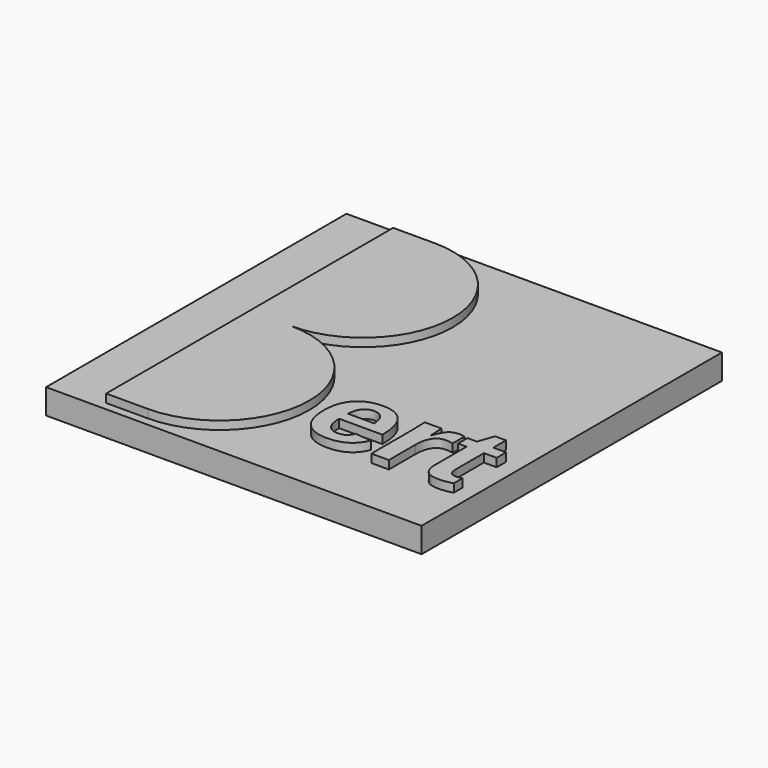
from build123d import *

# Parameters (mm, degrees)
F0_W         = 45
F0_H         = 45
F0_TEXT_SIZE = 15.2777777778
F1_DEPTH     = 3
F2_DEPTH     = 1


# Not quite as in the source:
# - Text() gives the source's letters only with a copy of the font that has no kerning and outlines rounded to 1/6400 em; it was checked with that copy


with BuildPart() as f1:
    # F0 (on Top) → F1 (new body)
    with BuildSketch(Plane.XY):
        with Locations((-17.3771874607, -9.7084985673)):
            Rectangle(F0_W, F0_H)
        with BuildLine():
            add(Edge.make_bspline(
                [(-8.1976327438, -23.1650957896), (-9.0570077438, -25.3588891923), (-11.6828757994, -25.3588891923)],
                knots=[0, 0, 0, 1, 1, 1], degree=2))
            add(Edge.make_bspline(
                [(-11.6828757994, -25.3588891923), (-13.5018862161, -25.3588891923), (-14.4794252786, -24.2798961368)],
                knots=[0, 0, 0, 1, 1, 1], degree=2))
            add(Edge.make_bspline(
                [(-14.4794252786, -24.2798961368), (-15.4569643411, -23.2009030812), (-15.4569643411, -21.1360159285)],
                knots=[0, 0, 0, 1, 1, 1], degree=2))
            add(Edge.make_bspline(
                [(-15.4569643411, -21.1360159285), (-15.4569643411, -19.1355819007), (-14.4651023619, -18.0613631507)],
                knots=[0, 0, 0, 1, 1, 1], degree=2))
            add(Edge.make_bspline(
                [(-14.4651023619, -18.0613631507), (-13.4732403827, -16.9871444007), (-11.6518428133, -16.9871444007)],
                knots=[0, 0, 0, 1, 1, 1], degree=2))
            add(Edge.make_bspline(
                [(-11.6518428133, -16.9871444007), (-9.9139955911, -16.9871444007), (-8.996135348, -18.1401391923)],
                knots=[0, 0, 0, 1, 1, 1], degree=2))
            add(Edge.make_bspline(
                [(-8.996135348, -18.1401391923), (-8.078275105, -19.293133984), (-8.078275105, -21.5155732201)],
                knots=[0, 0, 0, 1, 1, 1], degree=2))
            Line((-8.078275105, -21.5155732201), (-8.078275105, -21.5752520396))
            Line((-8.078275105, -21.5752520396), (-13.25600948, -21.5752520396))
            add(Edge.make_bspline(
                [(-13.25600948, -21.5752520396), (-13.25600948, -22.7545055118), (-12.8191605216, -23.3548744354)],
                knots=[0, 0, 0, 1, 1, 1], degree=2))
            add(Edge.make_bspline(
                [(-12.8191605216, -23.3548744354), (-12.3823115633, -23.955243359), (-11.5778410772, -23.955243359)],
                knots=[0, 0, 0, 1, 1, 1], degree=2))
            add(Edge.make_bspline(
                [(-11.5778410772, -23.955243359), (-10.4654278827, -23.955243359), (-10.1741952438, -22.9932207896)],
                knots=[0, 0, 0, 1, 1, 1], degree=2))
            Line((-10.1741952438, -22.9932207896), (-8.1976327438, -23.1650957896))
        make_face(mode=Mode.SUBTRACT)
        with BuildLine():
            Line((-4.3948983688, -25.2084985673), (-6.4908185077, -25.2084985673))
            Line((-6.4908185077, -25.2084985673), (-6.4908185077, -19.0305471785))
            add(Edge.make_bspline(
                [(-6.4908185077, -19.0305471785), (-6.4908185077, -18.3669187062), (-6.50991573, -17.9229082896)],
                knots=[0, 0, 0, 1, 1, 1], degree=2))
            add(Edge.make_bspline(
                [(-6.50991573, -17.9229082896), (-6.5290129522, -17.4788978729), (-6.5504973272, -17.1375350257)],
                knots=[0, 0, 0, 1, 1, 1], degree=2))
            Line((-6.5504973272, -17.1375350257), (-4.5524504522, -17.1375350257))
            add(Edge.make_bspline(
                [(-4.5524504522, -17.1375350257), (-4.5285789244, -17.2712155812), (-4.4915780563, -17.9539412757)],
                knots=[0, 0, 0, 1, 1, 1], degree=2))
            add(Edge.make_bspline(
                [(-4.4915780563, -17.9539412757), (-4.4545771883, -18.6366669701), (-4.4545771883, -18.8610593312)],
                knots=[0, 0, 0, 1, 1, 1], degree=2))
            Line((-4.4545771883, -18.8610593312), (-4.4235442022, -18.8610593312))
            add(Edge.make_bspline(
                [(-4.4235442022, -18.8610593312), (-4.1179886466, -18.0088457896), (-3.8792733688, -17.6627086368)],
                knots=[0, 0, 0, 1, 1, 1], degree=2))
            add(Edge.make_bspline(
                [(-3.8792733688, -17.6627086368), (-3.6405580911, -17.316571484), (-3.3123245841, -17.1482772132)],
                knots=[0, 0, 0, 1, 1, 1], degree=2))
            add(Edge.make_bspline(
                [(-3.3123245841, -17.1482772132), (-2.9840910772, -16.9799829423), (-2.492337605, -16.9799829423)],
                knots=[0, 0, 0, 1, 1, 1], degree=2))
            add(Edge.make_bspline(
                [(-2.492337605, -16.9799829423), (-2.0889087855, -16.9799829423), (-1.8430320494, -17.0921791229)],
                knots=[0, 0, 0, 1, 1, 1], degree=2))
            Line((-1.8430320494, -17.0921791229), (-1.8430320494, -18.8443492618))
            add(Edge.make_bspline(
                [(-1.8430320494, -18.8443492618), (-2.3514955911, -18.7321530812), (-2.7382143411, -18.7321530812)],
                knots=[0, 0, 0, 1, 1, 1], degree=2))
            add(Edge.make_bspline(
                [(-2.7382143411, -18.7321530812), (-3.5212004522, -18.7321530812), (-3.9580494105, -19.3671357201)],
                knots=[0, 0, 0, 1, 1, 1], degree=2))
            add(Edge.make_bspline(
                [(-3.9580494105, -19.3671357201), (-4.3948983688, -20.002118359), (-4.3948983688, -21.248212109)],
                knots=[0, 0, 0, 1, 1, 1], degree=2))
            Line((-4.3948983688, -21.248212109), (-4.3948983688, -25.2084985673))
        make_face(mode=Mode.SUBTRACT)
        with BuildLine():
            add(Edge.make_bspline(
                [(3.2893464228, -25.0891409285), (2.51352177, -25.3421791229), (1.5228533673, -25.3421791229)],
                knots=[0, 0, 0, 1, 1, 1], degree=2))
            add(Edge.make_bspline(
                [(1.5228533673, -25.3421791229), (0.5966380895, -25.3421791229), (0.0965295825, -24.8384898868)],
                knots=[0, 0, 0, 1, 1, 1], degree=2))
            add(Edge.make_bspline(
                [(0.0965295825, -24.8384898868), (-0.4035789244, -24.3348006507), (-0.4035789244, -23.3130992618)],
                knots=[0, 0, 0, 1, 1, 1], degree=2))
            Line((-0.4035789244, -23.3130992618), (-0.4035789244, -18.5531166229))
            Line((-0.4035789244, -18.5531166229), (-1.4252803133, -18.5531166229))
            Line((-1.4252803133, -18.5531166229), (-1.4252803133, -17.1375350257))
            Line((-1.4252803133, -17.1375350257), (-0.2985442022, -17.1375350257))
            Line((-0.2985442022, -17.1375350257), (0.3579228117, -15.2421357201))
            Line((0.3579228117, -15.2421357201), (1.6708568395, -15.2421357201))
            Line((1.6708568395, -15.2421357201), (1.6708568395, -17.1375350257))
            Line((1.6708568395, -17.1375350257), (3.20102177, -17.1375350257))
            Line((3.20102177, -17.1375350257), (3.20102177, -18.5531166229))
            Line((3.20102177, -18.5531166229), (1.6708568395, -18.5531166229))
            Line((1.6708568395, -18.5531166229), (1.6708568395, -22.7473440535))
            add(Edge.make_bspline(
                [(1.6708568395, -22.7473440535), (1.6708568395, -23.3369707896), (1.8952492006, -23.6162676646)],
                knots=[0, 0, 0, 1, 1, 1], degree=2))
            add(Edge.make_bspline(
                [(1.8952492006, -23.6162676646), (2.1196415617, -23.8955645396), (2.5875235062, -23.8955645396)],
                knots=[0, 0, 0, 1, 1, 1], degree=2))
            add(Edge.make_bspline(
                [(2.5875235062, -23.8955645396), (2.835787395, -23.8955645396), (3.2893464228, -23.7905298173)],
                knots=[0, 0, 0, 1, 1, 1], degree=2))
            Line((3.2893464228, -23.7905298173), (3.2893464228, -25.0891409285))
        make_face(mode=Mode.SUBTRACT)
        with BuildLine():
            Line((-33.4771874607, -31.2084985673), (-33.4771874607, 11.7915014327))
            Line((-33.4771874607, 11.7915014327), (-28.4771874607, 11.7915014327))
            ThreePointArc((-28.4771874607, 11.7915014327), (-17.7271874607, 1.0415014327), (-28.4771874607, -9.7084985673))
            ThreePointArc((-28.4771874607, -9.7084985673), (-17.7271874607, -20.4584985673), (-28.4771874607, -31.2084985673))
            Line((-28.4771874607, -31.2084985673), (-33.4771874607, -31.2084985673))
        make_face(mode=Mode.SUBTRACT)
        with BuildLine():
            Line((-28.4771874607, 11.7915014327), (-33.4771874607, 11.7915014327))
            Line((-33.4771874607, 11.7915014327), (-33.4771874607, -31.2084985673))
            Line((-33.4771874607, -31.2084985673), (-28.4771874607, -31.2084985673))
            ThreePointArc((-28.4771874607, -31.2084985673), (-17.7271874607, -20.4584985673), (-28.4771874607, -9.7084985673))
            ThreePointArc((-28.4771874607, -9.7084985673), (-17.7271874607, 1.0415014327), (-28.4771874607, 11.7915014327))
        make_face()
        with Locations((-16.0537525355, -25.2084985673)):
            Text('ert', F0_TEXT_SIZE, font='Arimo', font_style=FontStyle.BOLD, text_align=(TextAlign.LEFT, TextAlign.BOTTOM))
        with BuildLine():
            add(Edge.make_bspline(
                [(-10.5776240633, -18.7966062062), (-10.9882143411, -18.3072398868), (-11.6828757994, -18.3072398868)],
                knots=[0, 0, 0, 1, 1, 1], degree=2))
            add(Edge.make_bspline(
                [(-11.6828757994, -18.3072398868), (-12.4205060077, -18.3072398868), (-12.8191605216, -18.8228648868)],
                knots=[0, 0, 0, 1, 1, 1], degree=2))
            add(Edge.make_bspline(
                [(-12.8191605216, -18.8228648868), (-13.2178150355, -19.3384898868), (-13.2416865633, -20.2623180118)],
                knots=[0, 0, 0, 1, 1, 1], degree=2))
            Line((-13.2416865633, -20.2623180118), (-10.1073549661, -20.2623180118))
            add(Edge.make_bspline(
                [(-10.1073549661, -20.2623180118), (-10.1670337855, -19.2859725257), (-10.5776240633, -18.7966062062)],
                knots=[0, 0, 0, 1, 1, 1], degree=2))
        make_face()
    extrude(amount=-F1_DEPTH)

    # F0 (on Top) → F2 (join)
    with BuildSketch(Plane.XY):
        with BuildLine():
            Line((-28.4771874607, 11.7915014327), (-33.4771874607, 11.7915014327))
            Line((-33.4771874607, 11.7915014327), (-33.4771874607, -31.2084985673))
            Line((-33.4771874607, -31.2084985673), (-28.4771874607, -31.2084985673))
            ThreePointArc((-28.4771874607, -31.2084985673), (-17.7271874607, -20.4584985673), (-28.4771874607, -9.7084985673))
            ThreePointArc((-28.4771874607, -9.7084985673), (-17.7271874607, 1.0415014327), (-28.4771874607, 11.7915014327))
        make_face()
        with Locations((-16.0537525355, -25.2084985673)):
            Text('ert', F0_TEXT_SIZE, font='Arimo', font_style=FontStyle.BOLD, text_align=(TextAlign.LEFT, TextAlign.BOTTOM))
    extrude(amount=F2_DEPTH)


solid = f1.part
